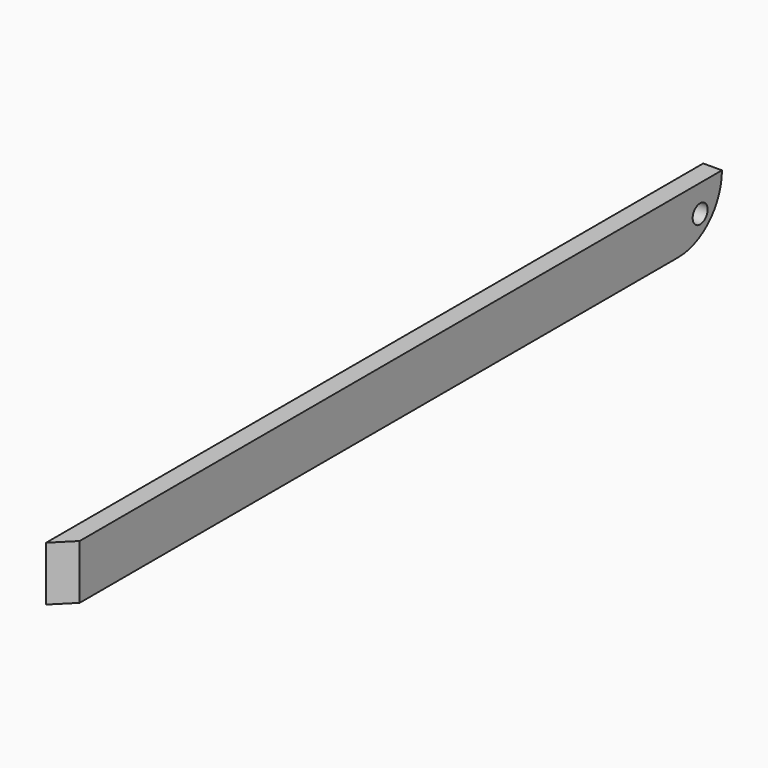
from build123d import *

# Parameters (mm, degrees)
F0_W     = 838.2
F0_H     = 55.5625
F1_DEPTH = 19.05
F2_R     = 55.56249
F3_R     = 9.525
F4_DEPTH = 25.4
F6_DEPTH = 55.5635


# Not quite as in the source:
# - a fillet or chamfer is up to 0.001 mm smaller than in the source, because OpenCascade refuses the exact size


with BuildPart() as f1:
    # F0 (on Right) → F1 (new body)
    with BuildSketch(Plane.YZ):
        with Locations((9.0487459762, 0)):
            Rectangle(F0_W, F0_H)
    extrude(amount=F1_DEPTH)

    # F2 (radius 55.5625 in the source; OpenCascade refuses exactly that, so slightly less here)
    f2_edges = [f1.edges().sort_by_distance(p)[0] for p in [
        (9.525, 428.148746, -27.78125),
    ]]
    fillet(f2_edges, radius=F2_R)

    # F3 (on face) → F4 (cut)
    with BuildSketch(Plane.YZ.offset(19.05)):
        with Locations((400.3674959762, 0)):
            Circle(F3_R)
    extrude(amount=-F4_DEPTH, mode=Mode.SUBTRACT)

    # F5 (on face) → F6 (cut, through all)
    with BuildSketch(Plane.XY.offset(27.78125)):
        Polygon((19.05, -391.0012540238), (0, -410.0512540238), (19.05, -410.0512540238), align=None)
    extrude(amount=-F6_DEPTH, mode=Mode.SUBTRACT)


solid = f1.part
